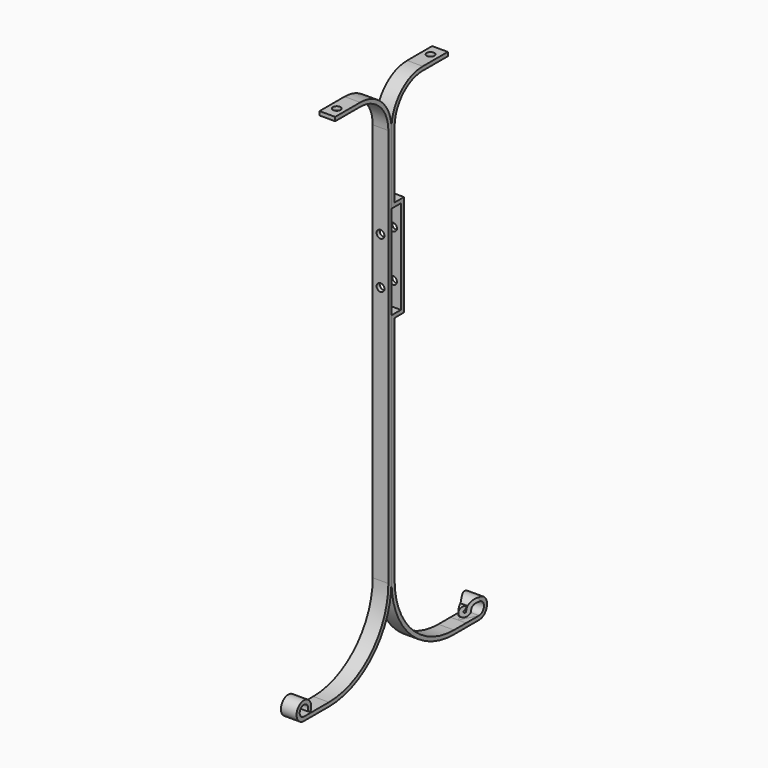
from build123d import *

# Parameters (mm, degrees)
F1_DEPTH  = 25.4
F2_R      = 6.35
F3_DEPTH  = 25.4009999233
F4_DEPTH  = 25.4
F5_R      = 6.35
F6_DEPTH  = 192.6798458016
F7_R      = 6.35
F8_DEPTH  = 25.4
F10_DEPTH = 37.846


# Not quite as in the source:
# - ends of sketch curves that miss each other by under 0.0002 mm in the source are joined


with BuildPart() as f1:
    # F0 (on Right) → F1 (new body)
    with BuildSketch(Plane.YZ):
        with BuildLine():
            ThreePointArc((63.5, 36.9650529042), (18.5987193947, 18.3663335095), (0, -26.5349470958))
            Line((0, -26.5349470958), (0, -140.8349470958))
            Line((0, -140.8349470958), (19.05, -140.8349470958))
            Line((19.05, -140.8349470958), (19.05, -293.2349470958))
            Line((19.05, -293.2349470958), (0, -293.2349470958))
            Line((0, -293.2349470958), (0, -674.2349470958))
            ThreePointArc((0, -674.2349470958), (37.1974387893, -764.0375083065), (127, -801.2349470958))
            Line((127, -801.2349470958), (177.8, -801.2349470958))
            ThreePointArc((177.8, -801.2349470958), (189.3975515729, -773.5690950337), (161.5385711193, -784.6947312355))
            ThreePointArc((161.5385711193, -784.6947312355), (158.2348270865, -785.7130978667), (160.2988376632, -782.9396981457))
            Line((160.2988376632, -782.9396981457), (162.3191535473, -776.9196629524))
            ThreePointArc((162.3191535473, -776.9196629524), (153.0483347508, -789.3768114543), (167.8876675483, -784.8026632189))
            ThreePointArc((167.8876675483, -784.8026632189), (184.8694148503, -778.0209095625), (177.8, -794.8849333338))
            Line((177.8, -794.8849333338), (127, -794.8849471726))
            ThreePointArc((127, -794.8849471726), (41.6875667956, -759.5473803002), (6.3499999233, -674.2349470958))
            Line((6.3499999233, -674.2349470958), (6.3499999233, -299.5849470191))
            Line((6.3499999233, -299.5849470191), (25.3999999233, -299.5849470191))
            Line((25.3999999233, -299.5849470191), (25.3999999233, -134.4849471726))
            Line((25.3999999233, -134.4849471726), (6.3499999233, -134.4849471726))
            Line((6.3499999233, -134.4849471726), (6.35, -26.5349470958))
            ThreePointArc((6.35, -26.5349470958), (23.0888474552, 13.876205449), (63.5, 30.6150529042))
            Line((63.5, 30.6150529042), (114.3, 30.6150529383))
            Line((114.3, 30.6150529383), (114.3, 36.9650529042))
            Line((114.3, 36.9650529042), (63.5, 36.9650529042))
        make_face()
    extrude(amount=F1_DEPTH)

    # F2 (on face) → F3 (cut, through all)
    with BuildSketch(Plane(origin=(0, 25.3999999233, 0), x_dir=(-1, 0, 0), z_dir=(0, 1, 0))):
        with Locations((-12.7, -178.9349470958)):
            Circle(F2_R)
        with Locations((-12.7, -255.1349470958)):
            Circle(F2_R)
    extrude(amount=-F3_DEPTH, mode=Mode.SUBTRACT)


with BuildPart() as f4:
    # F0 (on Right) → F4 (new body)
    with BuildSketch(Plane.YZ):
        with BuildLine():
            Line((0, -140.8349470958), (0, -26.5349470958))
            ThreePointArc((0, -26.5349470958), (-18.5987193947, 18.3663335095), (-63.5, 36.9650529042))
            Line((-63.5, 36.9650529042), (-114.3, 36.9650529042))
            Line((-114.3, 36.9650529042), (-114.3, 30.6150529383))
            Line((-114.3, 30.6150529383), (-63.5, 30.6150529042))
            ThreePointArc((-63.5, 30.6150529042), (-23.0888474552, 13.876205449), (-6.35, -26.5349470958))
            Line((-6.35, -26.5349470958), (-6.3499999233, -674.2349470958))
            ThreePointArc((-6.3499999233, -674.2349470958), (-41.6875667956, -759.5473803002), (-127, -794.8849471726))
            Line((-127, -794.8849471726), (-177.8, -794.8849471726))
            ThreePointArc((-177.8, -794.8849471726), (-182.2126311124, -779.0574998673), (-170.2477224413, -790.3189285424))
            Line((-170.2477224413, -790.3189285424), (-164.6247804165, -793.2693958282))
            ThreePointArc((-164.6247804165, -793.2693958282), (-185.4979935384, -773.6234288382), (-177.8, -801.2349470958))
            Line((-177.8, -801.2349470958), (-127, -801.2349470958))
            ThreePointArc((-127, -801.2349470958), (-37.1974387893, -764.0375083065), (0, -674.2349470958))
            Line((0, -674.2349470958), (0, -293.2349470958))
            Line((0, -293.2349470958), (0, -140.8349470958))
        make_face()
    extrude(amount=F4_DEPTH)

    # F5 (on face) → F6 (cut, through all)
    with BuildSketch(Plane(origin=(0, 0, 0), x_dir=(-1, 0, 0), z_dir=(0, 1, 0))):
        with Locations((-12.7, -178.9349470958)):
            Circle(F5_R)
        with Locations((-12.7, -255.1349470958)):
            Circle(F5_R)
    extrude(amount=-F6_DEPTH, mode=Mode.SUBTRACT)


with BuildPart() as f8_tool:
    # F7 (on face) → F8 (new body)
    with BuildSketch(Plane.XY.offset(36.9650529042)):
        with Locations((12.7, 95.25)):
            Circle(F7_R)
        with Locations((12.7, -95.25)):
            Circle(F7_R)
    extrude(amount=-F8_DEPTH)


with BuildPart() as f1_1:
    add(f1.part)

    # F8: cut by f8_tool
    add(f8_tool.part, mode=Mode.SUBTRACT)

    # F9 (on face) → F10 (cut)
    with BuildSketch(Plane.XY.offset(-794.8849471726)):
        Polygon((0, 151.5516016069), (12.7, 151.5516016069), (0, 177.8), align=None)
        Polygon((12.7, 151.5516016069), (25.4, 151.5516016069), (25.4, 177.8), align=None)
    extrude(amount=F10_DEPTH, mode=Mode.SUBTRACT)


with BuildPart() as f4_1:
    add(f4.part)

    # F8: cut by f8_tool
    add(f8_tool.part, mode=Mode.SUBTRACT)


solid = Compound([f1_1.part, f4_1.part])
